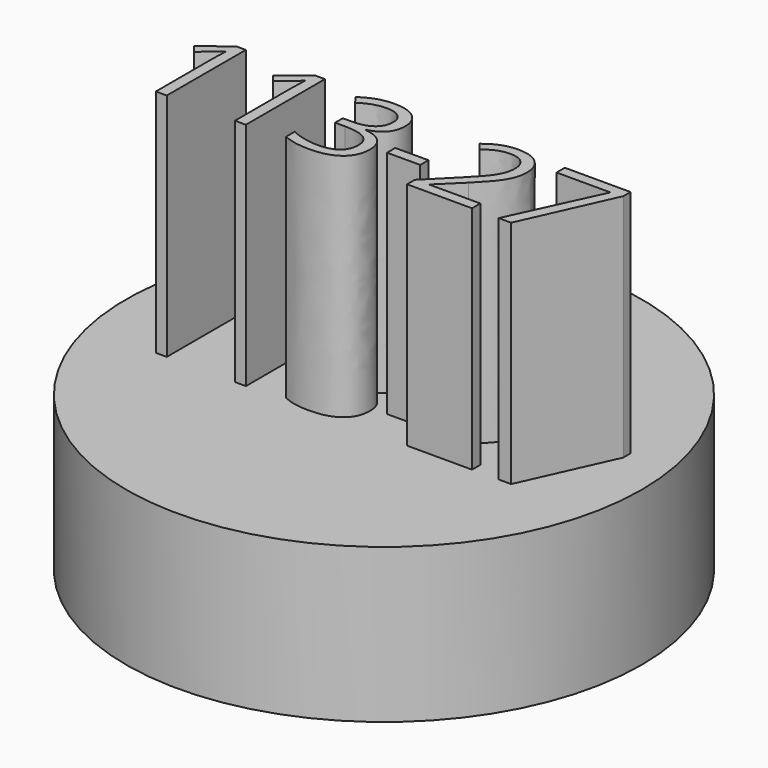
from build123d import *

# Parameters (mm, degrees)
F0_R         = 60.3281462918
F1_DEPTH     = 36.068
F2_TEXT_SIZE = 32.3784912729
F3_DEPTH     = 53.848


# Not quite as in the source:
# - Text() gives the source's letters only with a copy of the font that has no kerning and outlines rounded to 1/6400 em; it was checked with that copy


with BuildPart() as f1:
    # F0 (on Top) → F1 (new body)
    with BuildSketch(Plane.XY):
        Circle(F0_R)
    extrude(amount=F1_DEPTH)

    # F2 (on face) → F3 (join)
    with BuildSketch(Plane.XY.offset(36.068)):
        with Locations((-51.5897312871, -13.1672570569)):
            Text('113-27', F2_TEXT_SIZE, font='Open Sans', text_align=(TextAlign.LEFT, TextAlign.BOTTOM))
    extrude(amount=F3_DEPTH)


solid = f1.part
